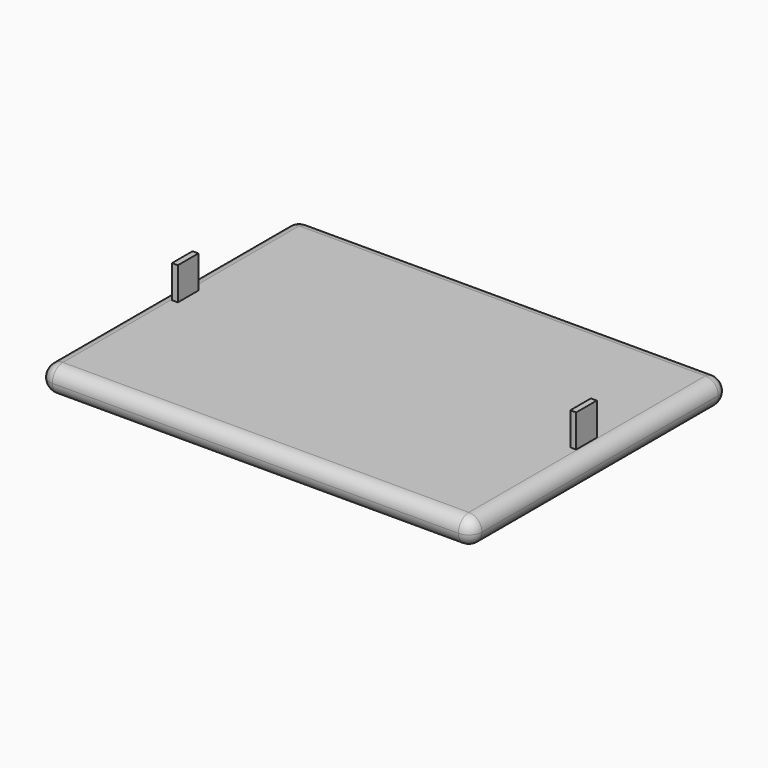
from build123d import *

# Parameters (mm, degrees)
F0_W     = 167.9448
F0_H     = 10.16
F1_DEPTH = 62.484
F2_W     = 2.2802874446
F2_H     = 9.9761183374
F3_DEPTH = 12.7
F4_R     = 5.07999


# Not quite as in the source:
# - a fillet or chamfer is up to 0.001 mm smaller than in the source, because OpenCascade refuses the exact size


with BuildPart() as f1:
    # F0 (on Front) → F1 (new body, symmetric)
    with BuildSketch(Plane.XZ):
        Rectangle(F0_W, F0_H)
    extrude(amount=F1_DEPTH, both=True)

    # F2 (on face) → F3 (join)
    with BuildSketch(Plane.XY.offset(5.08)):
        with Locations((-77.4024613202, 0.1807718072)):
            Rectangle(F2_W, F2_H)
        with Locations((77.4024613202, 0.1807718072)):
            Rectangle(F2_W, F2_H)
    extrude(amount=F3_DEPTH)

    # F4 (radius 5.08 in the source; OpenCascade refuses exactly that, so slightly less here)
    f4_edges = [f1.edges().sort_by_distance(p)[0] for p in [
        (0, -62.484, 5.08),
        (-83.9724, -62.484, 0),
        (0, -62.484, -5.08),
        (83.9724, -62.484, 0),
        (83.9724, 0, 5.08),
        (-83.9724, 0, 5.08),
        (0, 62.484, 5.08),
        (-83.9724, 0, -5.08),
        (0, 62.484, -5.08),
        (83.9724, 0, -5.08),
        (83.9724, 62.484, 0),
        (-83.9724, 62.484, 0),
    ]]
    fillet(f4_edges, radius=F4_R)


solid = f1.part
